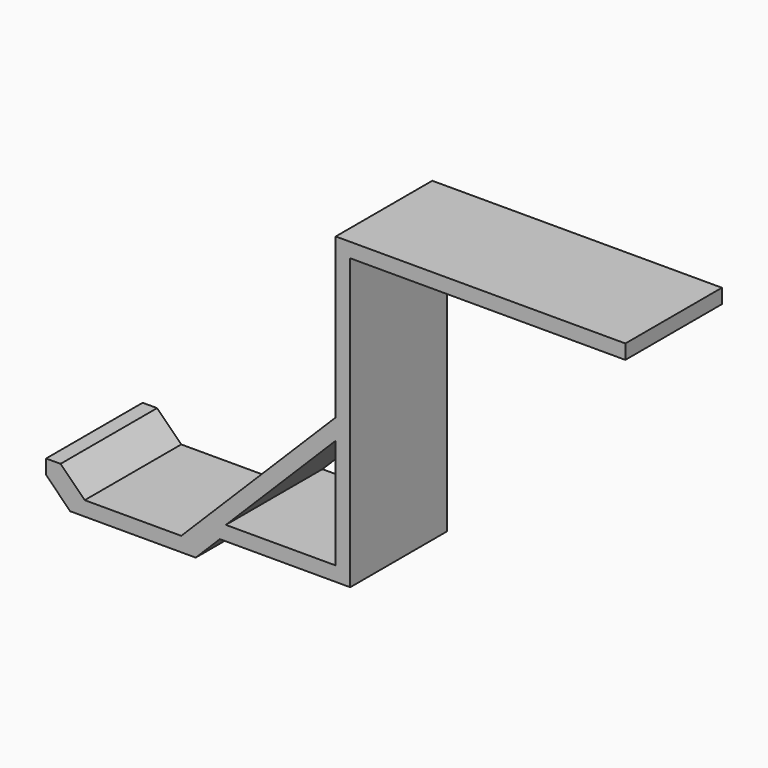
from build123d import *

# Parameters (mm, degrees)
F1_DEPTH = 25
F2_SIZE  = 4.99999


# Not quite as in the source:
# - a fillet or chamfer is up to 0.001 mm smaller than in the source, because OpenCascade refuses the exact size


with BuildPart() as f1:
    # F0 (on Front) → F1 (new body)
    with BuildSketch(Plane.XZ):
        Polygon((0, 22.7573593129), (0, 0), (-22.7573593129, 0), (-27, 0), (-32, 0), (-32, -5), (-57, -5), (-57, 0), (-60, 0), (-60, -8), (-29, -8), (-29, -3), (0, -3), (3, -3), (3, 57), (60, 57), (60, 60), (0, 60), (0, 27), align=None)
        Polygon((-22.7573593129, 0), (0, 22.7573593129), (0, 27), (-27, 0), align=None)
    extrude(amount=F1_DEPTH)

    # F2 (size 5 in the source; OpenCascade refuses exactly that, so slightly less here)
    f2_edges = [f1.edges().sort_by_distance(p)[0] for p in [
        (-57, -12.5, -5),
        (-60, -12.5, -8),
        (-29, -12.5, -3),
        (-32, -12.5, 0),
    ]]
    chamfer(f2_edges, length=F2_SIZE)


solid = f1.part
